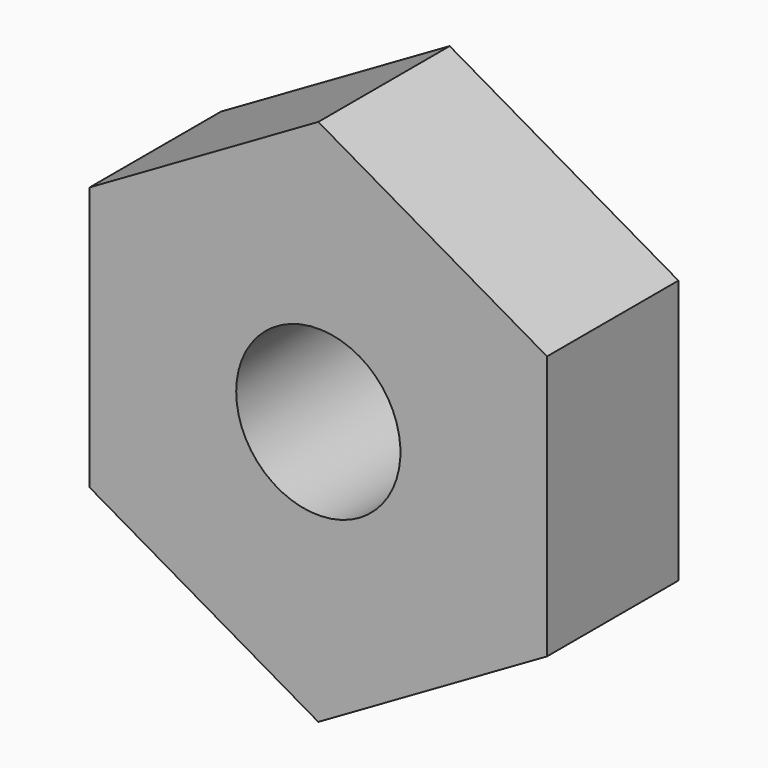
from build123d import *

# Parameters (mm, degrees)
F1_DEPTH = 5.842
F2_D     = 5.842


# Not quite as in the source:
# - a feature names something its author has since deleted; it is built from what else it names


with BuildPart() as f1:
    # F0 (on Front) → F1 (new body)
    with BuildSketch(Plane.XZ):
        Polygon((58.9488451577, 9.395414032), (50.8121779269, 4.697707016), (50.8121779269, -4.697707016), (58.9488451577, -9.395414032), (67.0855123886, -4.697707016), (67.0855123886, 4.697707016), align=None)
    extrude(amount=F1_DEPTH)

    # F2 (through all)
    with Locations(Plane(origin=(0, 0, 0), x_dir=(1, 0, 0), z_dir=(0, 1, 0))):
        with Locations((58.9488451577, 0)):
            Hole(F2_D / 2)


solid = f1.part
